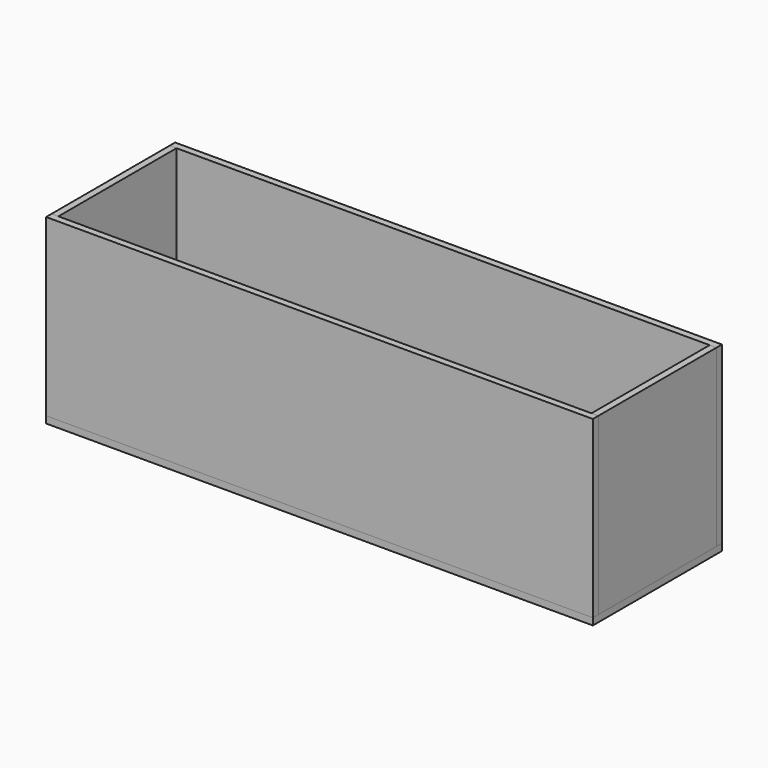
from build123d import *

# Parameters (mm, degrees)
F0_W     = 2000
F0_H     = 640
F1_DEPTH = 25
F2_W     = 2000
F2_H     = 590
F3_DEPTH = 25
F5_W     = 540
F5_H     = 640
F6_DEPTH = 25
F7_W     = 540
F7_H     = 640
F8_DEPTH = 25


# Not quite as in the source:
# - a feature of the source that left no trace in its solid (it failed there, or was rolled back) is left out
# - a pattern or mirror of a feature is missing from the dataset's text; its kind, count and spacing are read off the source's solid


with BuildPart() as f1:
    # F0 (on Front) → F1 (new body)
    with BuildSketch(Plane.XZ):
        with Locations((1000, 320)):
            Rectangle(F0_W, F0_H)
    extrude(amount=F1_DEPTH)


with BuildPart() as f1_copies_1:
    # F1_copies: instance of F1
    add(f1.part.mirror(Plane(origin=(0, -295, 0), x_dir=(0, 0, -1), z_dir=(0, -1, 0))))


with BuildPart() as f3:
    # F2 (on Top) → F3 (new body)
    with BuildSketch(Plane.XY):
        with Locations((1000, -295)):
            Rectangle(F2_W, F2_H)
    extrude(amount=-F3_DEPTH)


with BuildPart() as f6:
    # F5 (on Right) → F6 (new body)
    with BuildSketch(Plane.YZ):
        with Locations((-295, 320)):
            Rectangle(F5_W, F5_H)
    extrude(amount=F6_DEPTH)


with BuildPart() as f8:
    # F7 (on face) → F8 (new body)
    with BuildSketch(Plane.YZ.offset(2000)):
        with Locations((-295, 320)):
            Rectangle(F7_W, F7_H)
    extrude(amount=-F8_DEPTH)


solid = Compound([f1.part, f1_copies_1.part, f3.part, f6.part, f8.part])
